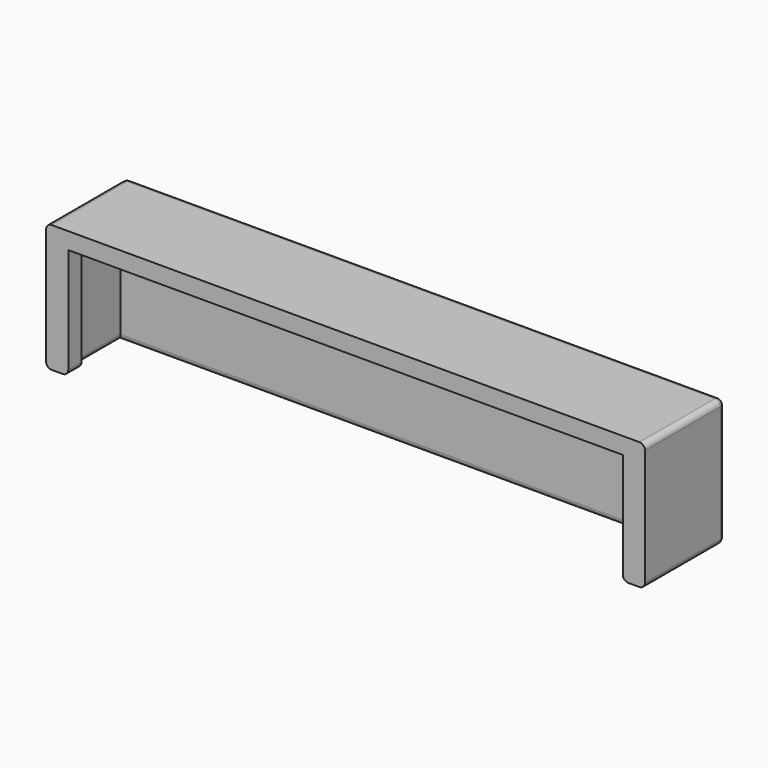
from build123d import *

# Parameters (mm, degrees)
F0_W     = 1
F0_H     = 20
F0_W_2   = 100
F1_DEPTH = 18
F2_DEPTH = 13
F3_DEPTH = 3
F4_R     = 0.9999


# Not quite as in the source:
# - a fillet or chamfer is up to 0.001 mm smaller than in the source, because OpenCascade refuses the exact size


with BuildPart() as f1:
    # F0 (on Front) → F1 (new body)
    with BuildSketch(Plane.XZ):
        Polygon((51, 20), (51, 0), (54, 0), (54, 23), (-54, 23), (-54, 0), (-51, 0), (-51, 20), (-50, 20), (50, 20), align=None)
        with Locations((-50.5, 10)):
            Rectangle(F0_W, F0_H)
        with Locations((0, 10)):
            Rectangle(F0_W_2, F0_H)
        with Locations((50.5, 10)):
            Rectangle(F0_W, F0_H)
    extrude(amount=-F1_DEPTH)

    # F0 (on Front) → F2 (cut)
    with BuildSketch(Plane.XZ):
        with Locations((-50.5, 10)):
            Rectangle(F0_W, F0_H)
        with Locations((0, 10)):
            Rectangle(F0_W_2, F0_H)
        with Locations((50.5, 10)):
            Rectangle(F0_W, F0_H)
    extrude(amount=-F2_DEPTH, mode=Mode.SUBTRACT)

    # F0 (on Front) → F3 (join)
    with BuildSketch(Plane.XZ):
        with Locations((-50.5, 10)):
            Rectangle(F0_W, F0_H)
        with Locations((50.5, 10)):
            Rectangle(F0_W, F0_H)
    extrude(amount=-F3_DEPTH)

    # F4 (radius 1 in the source; OpenCascade refuses exactly that, so slightly less here)
    f4_edges = [f1.edges().sort_by_distance(p)[0] for p in [
        (-54, 18, 11.5),
        (54, 18, 11.5),
        (0, 18, 0),
        (54, 9, 0),
        (-54, 9, 0),
        (-54, 9, 23),
        (0, 18, 23),
        (54, 9, 23),
        (0, 13, 0),
        (51, 8, 0),
        (-51, 8, 0),
        (-50, 1.5, 0),
        (50, 1.5, 0),
    ]]
    fillet(f4_edges, radius=F4_R)


solid = f1.part
